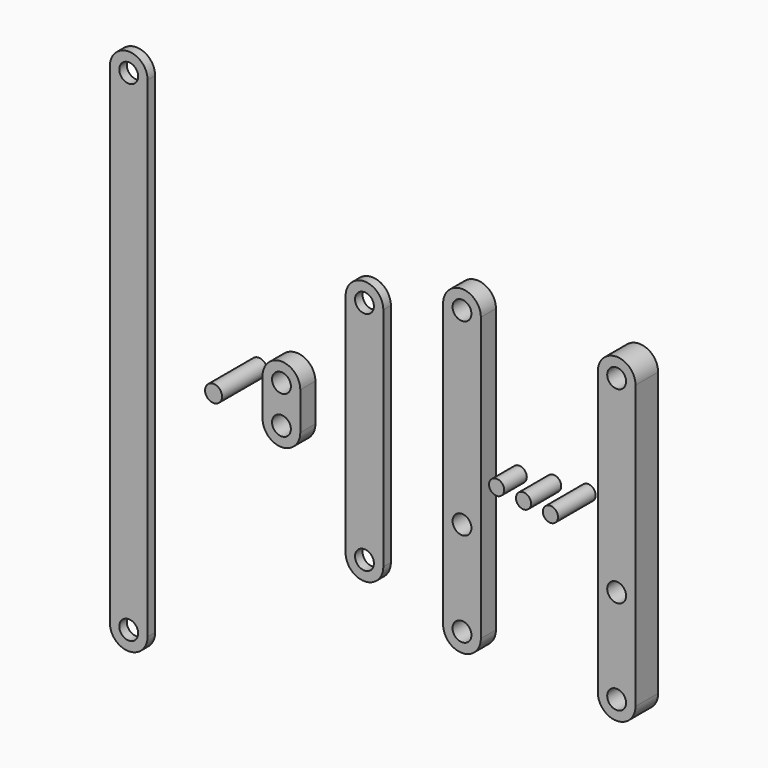
from build123d import *

# Parameters (mm, degrees)
F2_R      = 2.5
F3_DEPTH  = 2.5
F4_R      = 2.5
F5_DEPTH  = 1.25
F6_R      = 2.5
F7_DEPTH  = 2.5
F8_R      = 2
F9_DEPTH  = 3.75
F10_R     = 2
F11_DEPTH = 5
F12_R     = 2.5
F13_DEPTH = 3.75
F14_R     = 2
F15_DEPTH = 6.25
F16_R     = 2.25
F17_DEPTH = 7.5
F18_R     = 2.5
F19_DEPTH = 2.5


with BuildPart() as f3:
    # F2 (on Front) → F3 (new body, symmetric)
    with BuildSketch(Plane.XZ):
        with BuildLine():
            Line((5, 0), (5, 37.5))
            ThreePointArc((5, 37.5), (0, 42.5), (-5, 37.5))
            Line((-5, 37.5), (-5, 0))
            Line((-5, 0), (-5, -37.5))
            ThreePointArc((-5, -37.5), (0, -42.5), (5, -37.5))
            Line((5, -37.5), (5, 0))
        make_face()
        with Locations((0, -37.5)):
            Circle(F2_R, mode=Mode.SUBTRACT)
        with Locations((0, -12.5)):
            Circle(F2_R, mode=Mode.SUBTRACT)
        with Locations((0, 37.5)):
            Circle(F2_R, mode=Mode.SUBTRACT)
    extrude(amount=F3_DEPTH, both=True)


with BuildPart() as f5:
    # F4 (on Front) → F5 (new body, symmetric)
    with BuildSketch(Plane.XZ):
        with BuildLine():
            Line((-21.8589119613, 0), (-21.8589119613, 30))
            ThreePointArc((-21.8589119613, 30), (-26.8589119613, 35), (-31.8589119613, 30))
            Line((-31.8589119613, 30), (-31.8589119613, 0))
            Line((-31.8589119613, 0), (-31.8589119613, -30))
            ThreePointArc((-31.8589119613, -30), (-26.8589119613, -35), (-21.8589119613, -30))
            Line((-21.8589119613, -30), (-21.8589119613, 0))
        make_face()
        with Locations((-26.8589119613, -30)):
            Circle(F4_R, mode=Mode.SUBTRACT)
        with Locations((-26.8589119613, 30)):
            Circle(F4_R, mode=Mode.SUBTRACT)
    extrude(amount=F5_DEPTH, both=True)


with BuildPart() as f7:
    # F6 (on Front) → F7 (new body, symmetric)
    with BuildSketch(Plane.XZ):
        with BuildLine():
            Line((-42.8727790713, 0), (-42.8727790713, 5))
            ThreePointArc((-42.8727790713, 5), (-47.8727790713, 10), (-52.8727790713, 5))
            Line((-52.8727790713, 5), (-52.8727790713, 0))
            Line((-52.8727790713, 0), (-52.8727790713, -5))
            ThreePointArc((-52.8727790713, -5), (-47.8727790713, -10), (-42.8727790713, -5))
            Line((-42.8727790713, -5), (-42.8727790713, 0))
        make_face()
        with Locations((-47.8727790713, -5)):
            Circle(F6_R, mode=Mode.SUBTRACT)
        with Locations((-47.8727790713, 5)):
            Circle(F6_R, mode=Mode.SUBTRACT)
    extrude(amount=F7_DEPTH, both=True)


with BuildPart() as f9:
    # F8 (on Front) → F9 (new body, symmetric)
    with BuildSketch(Plane.XZ):
        with Locations((10.1797801788, 0)):
            Circle(F8_R)
    extrude(amount=F9_DEPTH, both=True)


with BuildPart() as f11:
    # F10 (on Front) → F11 (new body, symmetric)
    with BuildSketch(Plane.XZ):
        with Locations((18.3083742857, 0)):
            Circle(F10_R)
    extrude(amount=F11_DEPTH, both=True)


with BuildPart() as f13:
    # F12 (on face) → F13 (new body, symmetric)
    with BuildSketch(Plane.XZ.offset(2.5)):
        with BuildLine():
            Line((49.0088026483, 0), (49.0088026483, 37.5))
            ThreePointArc((49.0088026483, 37.5), (44.0088026483, 42.5), (39.0088026483, 37.5))
            Line((39.0088026483, 37.5), (39.0088026483, 0))
            Line((39.0088026483, 0), (39.0088026483, -37.5))
            ThreePointArc((39.0088026483, -37.5), (44.0088026483, -42.5), (49.0088026483, -37.5))
            Line((49.0088026483, -37.5), (49.0088026483, 0))
        make_face()
        with Locations((44.0088026483, -37.5)):
            Circle(F12_R, mode=Mode.SUBTRACT)
        with Locations((44.0088026483, -12.5)):
            Circle(F12_R, mode=Mode.SUBTRACT)
        with Locations((44.0088026483, 37.5)):
            Circle(F12_R, mode=Mode.SUBTRACT)
    extrude(amount=F13_DEPTH, both=True)


with BuildPart() as f15:
    # F14 (on Front) → F15 (new body, symmetric)
    with BuildSketch(Plane.XZ):
        with Locations((26.4492426068, 0)):
            Circle(F14_R)
    extrude(amount=F15_DEPTH, both=True)


with BuildPart() as f17:
    # F16 (on Front) → F17 (new body, symmetric)
    with BuildSketch(Plane.XZ):
        with Locations((-61.8761591613, 0)):
            Circle(F16_R)
    extrude(amount=F17_DEPTH, both=True)


with BuildPart() as f19:
    # F18 (on face) → F19 (new body)
    with BuildSketch(Plane.XZ.offset(1.25)):
        with BuildLine():
            Line((-82.3671596532, 0), (-82.3671596532, 65))
            ThreePointArc((-82.3671596532, 65), (-87.3671596532, 70), (-92.3671596532, 65))
            Line((-92.3671596532, 65), (-92.3671596532, 0))
            Line((-92.3671596532, 0), (-92.3671596532, -65))
            ThreePointArc((-92.3671596532, -65), (-87.3671596532, -70), (-82.3671596532, -65))
            Line((-82.3671596532, -65), (-82.3671596532, 0))
        make_face()
        with Locations((-87.3671596532, -65)):
            Circle(F18_R, mode=Mode.SUBTRACT)
        with Locations((-87.3671596532, 65)):
            Circle(F18_R, mode=Mode.SUBTRACT)
    extrude(amount=F19_DEPTH)


solid = Compound([f3.part, f5.part, f7.part, f9.part, f11.part, f13.part, f15.part, f17.part, f19.part])
